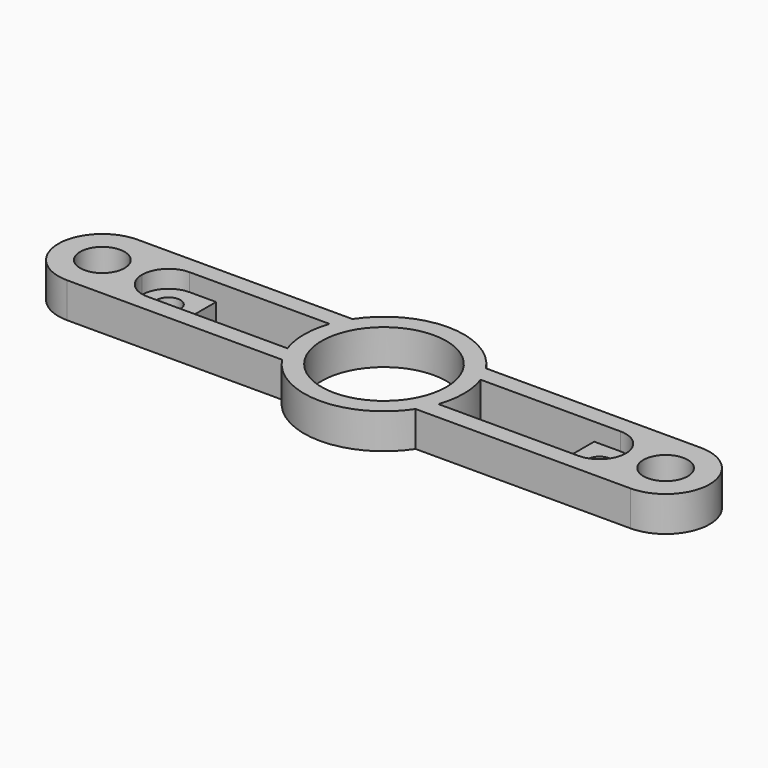
from build123d import *

# Parameters (mm, degrees)
F0_R     = 4
F0_R_2   = 11.2530001
F1_DEPTH = 6.35
F2_R     = 2.15265
F3_DEPTH = 6.35
F4_W     = 9.525
F4_H     = 9.525
F5_DEPTH = 3.175
F6_R     = 4.76249


# Not quite as in the source:
# - a fillet or chamfer is up to 0.001 mm smaller than in the source, because OpenCascade refuses the exact size


with BuildPart() as f1:
    # F0 (on Top) → F1 (new body)
    with BuildSketch(Plane.XY):
        with BuildLine():
            Line((-12.0483725306, 7.9375), (-50.8, 7.9375))
            ThreePointArc((-50.8, 7.9375), (-58.7375, 0), (-50.8, -7.9375))
            Line((-50.8, -7.9375), (-12.0483725306, -7.9375))
            ThreePointArc((-12.0483725306, -7.9375), (0, -14.4280001), (12.0483725306, -7.9375))
            Line((12.0483725306, -7.9375), (50.8, -7.9375))
            ThreePointArc((50.8, -7.9375), (58.7375, 0), (50.8, 7.9375))
            Line((50.8, 7.9375), (12.0483725306, 7.9375))
            ThreePointArc((12.0483725306, 7.9375), (0, 14.4280001), (-12.0483725306, 7.9375))
        make_face()
        with Locations((-50.8, 0)):
            Circle(F0_R, mode=Mode.SUBTRACT)
        Circle(F0_R_2, mode=Mode.SUBTRACT)
        with Locations((50.8, 0)):
            Circle(F0_R, mode=Mode.SUBTRACT)
    extrude(amount=F1_DEPTH)

    # F2 (on face) → F3 (cut, through all)
    with BuildSketch(Plane.XY.offset(6.35)):
        with BuildLine():
            ThreePointArc((-13.6193164526, -4.7625), (-14.4280001, 0), (-13.6193164526, 4.7625))
            Line((-13.6193164526, 4.7625), (-34.1, 4.7625))
            Line((-34.1, 4.7625), (-34.1, -4.7625))
            Line((-34.1, -4.7625), (-13.6193164526, -4.7625))
        make_face()
        with BuildLine():
            Line((34.1, 4.7625), (13.6193164526, 4.7625))
            ThreePointArc((13.6193164526, 4.7625), (14.4280001, 0), (13.6193164526, -4.7625))
            Line((13.6193164526, -4.7625), (34.1, -4.7625))
            Line((34.1, -4.7625), (34.1, 4.7625))
        make_face()
        with Locations((-38.8625, 0)):
            Circle(F2_R)
        with Locations((38.8625, 0)):
            Circle(F2_R)
    extrude(amount=-F3_DEPTH, mode=Mode.SUBTRACT)

    # F4 (on face) → F5 (cut)
    with BuildSketch(Plane.XY.offset(6.35)):
        with Locations((-38.8625, 0)):
            Rectangle(F4_W, F4_H)
        with Locations((38.8625, 0)):
            Rectangle(F4_W, F4_H)
    extrude(amount=-F5_DEPTH, mode=Mode.SUBTRACT)

    # F6 (radius 4.7625 in the source; OpenCascade refuses exactly that, so slightly less here)
    f6_edges = [f1.edges().sort_by_distance(p)[0] for p in [
        (-43.625, 4.7625, 4.7625),
        (-43.625, -4.7625, 4.7625),
        (43.625, 4.7625, 4.7625),
        (43.625, -4.7625, 4.7625),
    ]]
    fillet(f6_edges, radius=F6_R)


solid = f1.part
